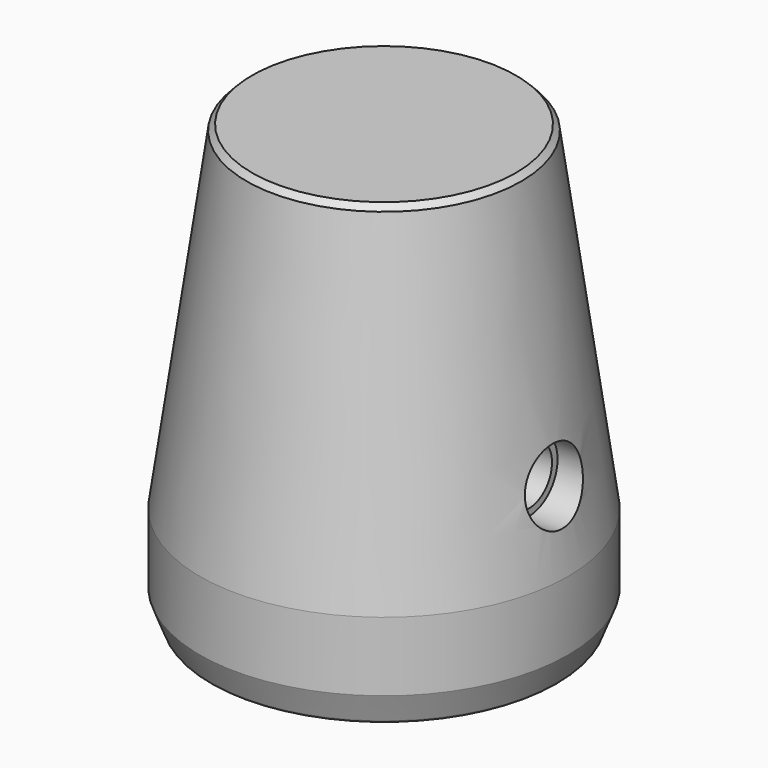
from build123d import *

# Parameters (mm, degrees)
F3_SIZE        = 1
F4_SIZE2       = 0.2
F4_SIZE        = 0.25
F5_R           = 0.1524
F8_D           = 2.5
F8_DEPTH       = 8
F8_START       = 0.6998646
F8_CBORE_D     = 3.1
F8_CBORE_DEPTH = 1
F8_TIP         = 0.7510757738
F9_R           = 2.78
F10_DEPTH      = 2.15
F12_DEPTH      = 2.5


with BuildPart() as f2:
    # F1 (on Front) → F2 (revolve)
    with BuildSketch(Plane.XZ):
        Polygon((6.8, 4.2), (6.8, 0), (7.5, 0), (8, 1.3), (8, 4.3), (5.9340497299, 19), (0, 19), (0, 18), (1.61, 18), (1.61, 4.2), align=None)
    revolve(axis=Axis((0, 0, 11.6), (0, 0, 1)))

    # F3
    f3_edges = [f2.edges().sort_by_distance(p)[0] for p in [
        (-1.61, 0, 18),
    ]]
    chamfer(f3_edges, length=F3_SIZE)

    # F4
    f4_edges = [f2.edges().sort_by_distance(p)[0] for p in [
        (-5.93405, 0, 19),
    ]]
    chamfer(f4_edges, length=F4_SIZE, length2=F4_SIZE2)

    # F5
    f5_edges = [f2.edges().sort_by_distance(p)[0] for p in [
        (-6.8, 0, 0),
        (-7.5, 0, 0),
        (-6.8, 0, 4.2),
        (-1.61, 0, 4.2),
    ]]
    fillet(f5_edges, radius=F5_R)

    # F8
    # its depths count from where the whole tool has entered the part; down to there all is cleared
    with Locations(Plane.YZ.offset(8).offset(-F8_START)):
        with Locations((0, 7.6)):
            CounterBoreHole(F8_D / 2, F8_CBORE_D / 2, F8_CBORE_DEPTH, depth=F8_DEPTH)
            with Locations((0, 0, -(F8_DEPTH + F8_TIP / 2))):  # 118° drill point
                Cone(0, F8_D / 2, F8_TIP, mode=Mode.SUBTRACT)


with BuildPart() as f10:
    # F9 (on Top) → F10 (new body)
    with BuildSketch(Plane.XY):
        Polygon((-2.3036275741, -3.99), (2.3036275741, -3.99), (4.6072551481, 0), (2.3036275741, 3.99), (-2.3036275741, 3.99), (-4.6072551481, 0), align=None)
        Circle(F9_R, mode=Mode.SUBTRACT)
    extrude(amount=F10_DEPTH)


with BuildPart() as f12:
    # F11 (on Top) → F12 (new body)
    with BuildSketch(Plane.XY):
        Polygon((-3.1754264805, -5.5), (3.1754264805, -5.5), (6.3508529611, 0), (3.1754264805, 5.5), (-3.1754264805, 5.5), (-6.3508529611, 0), align=None)
    extrude(amount=F12_DEPTH)


solid = Compound([f2.part, f10.part, f12.part])
